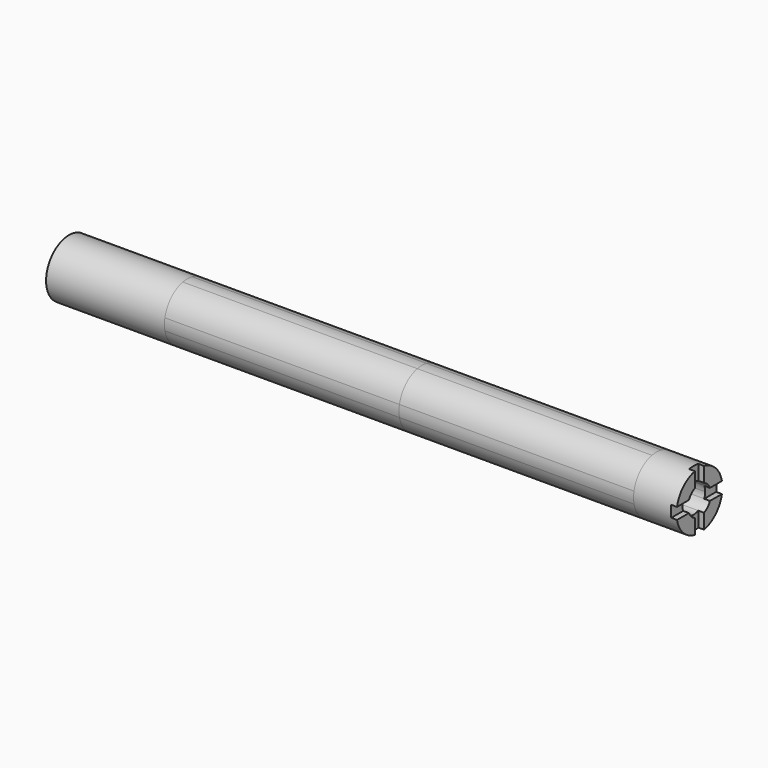
from build123d import *
from build123d import SkipClean  # not in build123d's __all__

# Parameters (mm, degrees)
F1_DEPTH  = 103.9495
F3_R      = 12.7
F4_DEPTH  = 19.05
F6_DEPTH  = 25.4
F8_DEPTH  = 2.54
F9_R      = 12.7
F10_DEPTH = 52.451


# Not quite as in the source:
# - after a boolean that leaves OpenCascade's solid faulty, fix() repairs it


with BuildPart() as f1:
    # F0 (on Right) → F1 (new body, symmetric)
    with BuildSketch(Plane.YZ):
        with BuildLine():
            ThreePointArc((12.4434078933, -2.54), (12.6356891432, -1.2764638175), (12.7, 0))
            ThreePointArc((12.7, 0), (12.6356891432, 1.2764638175), (12.4434078933, 2.54))
            Line((12.4434078933, 2.54), (5.8198711326, 2.54))
            ThreePointArc((5.8198711326, 2.54), (6.2160550871, 1.2973662374), (6.35, 0))
            ThreePointArc((6.35, 0), (6.2160550871, -1.2973662374), (5.8198711326, -2.54))
            Line((5.8198711326, -2.54), (12.4434078933, -2.54))
        make_face()
        with BuildLine():
            Line((5.8198711326, 2.54), (12.4434078933, 2.54))
            ThreePointArc((12.4434078933, 2.54), (8.9802561211, 8.9802561211), (2.54, 12.4434078933))
            Line((2.54, 12.4434078933), (2.54, 5.8198711326))
            ThreePointArc((2.54, 5.8198711326), (4.4901280605, 4.4901280605), (5.8198711326, 2.54))
        make_face()
        with BuildLine():
            ThreePointArc((2.54, -12.4434078933), (8.9802561211, -8.9802561211), (12.4434078933, -2.54))
            Line((12.4434078933, -2.54), (5.8198711326, -2.54))
            ThreePointArc((5.8198711326, -2.54), (4.4901280605, -4.4901280605), (2.54, -5.8198711326))
            Line((2.54, -5.8198711326), (2.54, -12.4434078933))
        make_face()
        with BuildLine():
            Line((2.54, 5.8198711326), (2.54, 12.4434078933))
            ThreePointArc((2.54, 12.4434078933), (0, 12.7), (-2.54, 12.4434078933))
            Line((-2.54, 12.4434078933), (-2.54, 5.8198711326))
            ThreePointArc((-2.54, 5.8198711326), (0, 6.35), (2.54, 5.8198711326))
        make_face()
        with BuildLine():
            ThreePointArc((-2.54, -12.4434078933), (0, -12.7), (2.54, -12.4434078933))
            Line((2.54, -12.4434078933), (2.54, -5.8198711326))
            ThreePointArc((2.54, -5.8198711326), (0, -6.35), (-2.54, -5.8198711326))
            Line((-2.54, -5.8198711326), (-2.54, -12.4434078933))
        make_face()
        with BuildLine():
            Line((-2.54, 5.8198711326), (-2.54, 12.4434078933))
            ThreePointArc((-2.54, 12.4434078933), (-8.9802561211, 8.9802561211), (-12.4434078933, 2.54))
            Line((-12.4434078933, 2.54), (-5.8198711326, 2.54))
            ThreePointArc((-5.8198711326, 2.54), (-4.4901280605, 4.4901280605), (-2.54, 5.8198711326))
        make_face()
        with BuildLine():
            ThreePointArc((-12.4434078933, -2.54), (-8.9802561211, -8.9802561211), (-2.54, -12.4434078933))
            Line((-2.54, -12.4434078933), (-2.54, -5.8198711326))
            ThreePointArc((-2.54, -5.8198711326), (-4.4901280605, -4.4901280605), (-5.8198711326, -2.54))
            Line((-5.8198711326, -2.54), (-12.4434078933, -2.54))
        make_face()
        with BuildLine():
            Line((-5.8198711326, 2.54), (-12.4434078933, 2.54))
            ThreePointArc((-12.4434078933, 2.54), (-12.7, 0), (-12.4434078933, -2.54))
            Line((-12.4434078933, -2.54), (-5.8198711326, -2.54))
            ThreePointArc((-5.8198711326, -2.54), (-6.35, 0), (-5.8198711326, 2.54))
        make_face()
        with BuildLine():
            ThreePointArc((6.35, 0), (6.2160550871, 1.2973662374), (5.8198711326, 2.54))
            ThreePointArc((5.8198711326, 2.54), (4.4901280605, 4.4901280605), (2.54, 5.8198711326))
            ThreePointArc((2.54, 5.8198711326), (0, 6.35), (-2.54, 5.8198711326))
            ThreePointArc((-2.54, 5.8198711326), (-4.4901280605, 4.4901280605), (-5.8198711326, 2.54))
            ThreePointArc((-5.8198711326, 2.54), (-6.35, 0), (-5.8198711326, -2.54))
            ThreePointArc((-5.8198711326, -2.54), (-4.4901280605, -4.4901280605), (-2.54, -5.8198711326))
            ThreePointArc((-2.54, -5.8198711326), (0, -6.35), (2.54, -5.8198711326))
            ThreePointArc((2.54, -5.8198711326), (4.4901280605, -4.4901280605), (5.8198711326, -2.54))
            ThreePointArc((5.8198711326, -2.54), (6.2160550871, -1.2973662374), (6.35, 0))
        make_face()
    extrude(amount=F1_DEPTH, both=True)

    # F3 (on face) → F4 (join)
    with BuildSketch(Plane.YZ.offset(103.9495)):
        Circle(F3_R)
    with SkipClean():  # cleaning this boolean's faces spoils the solid; the shape is the same uncleaned
        extrude(amount=F4_DEPTH)

    # F5 (on face) → F6 (cut)
    with BuildSketch(Plane.YZ.offset(122.9995)):
        with BuildLine():
            ThreePointArc((5.8198711326, -2.54), (6.2160550871, -1.2973662374), (6.35, 0))
            ThreePointArc((6.35, 0), (6.2160550871, 1.2973662374), (5.8198711326, 2.54))
            ThreePointArc((5.8198711326, 2.54), (4.4901280605, 4.4901280605), (2.54, 5.8198711326))
            ThreePointArc((2.54, 5.8198711326), (0, 6.35), (-2.54, 5.8198711326))
            ThreePointArc((-2.54, 5.8198711326), (-4.4901280605, 4.4901280605), (-5.8198711326, 2.54))
            ThreePointArc((-5.8198711326, 2.54), (-6.35, 0), (-5.8198711326, -2.54))
            ThreePointArc((-5.8198711326, -2.54), (-4.4901280605, -4.4901280605), (-2.54, -5.8198711326))
            ThreePointArc((-2.54, -5.8198711326), (0, -6.35), (2.54, -5.8198711326))
            ThreePointArc((2.54, -5.8198711326), (4.4901280605, -4.4901280605), (5.8198711326, -2.54))
        make_face()
    extrude(amount=-F6_DEPTH, mode=Mode.SUBTRACT)

    add(f1.part.fix(), mode=Mode.REPLACE)

    # F7 (on face) → F8 (cut)
    with BuildSketch(Plane.YZ.offset(122.9995)):
        with BuildLine():
            ThreePointArc((2.54, 12.4434078933), (0, 12.7), (-2.54, 12.4434078933))
            Line((-2.54, 12.4434078933), (-2.54, 5.8198711326))
            ThreePointArc((-2.54, 5.8198711326), (0, 6.35), (2.54, 5.8198711326))
            Line((2.54, 5.8198711326), (2.54, 12.4434078933))
        make_face()
        with BuildLine():
            ThreePointArc((12.7, 0), (12.6356891432, 1.2764638175), (12.4434078933, 2.54))
            Line((12.4434078933, 2.54), (5.8198711326, 2.54))
            ThreePointArc((5.8198711326, 2.54), (6.2160550871, 1.2973662374), (6.35, 0))
            ThreePointArc((6.35, 0), (6.2160550871, -1.2973662374), (5.8198711326, -2.54))
            Line((5.8198711326, -2.54), (12.4434078933, -2.54))
            ThreePointArc((12.4434078933, -2.54), (12.6356891432, -1.2764638175), (12.7, 0))
        make_face()
        with BuildLine():
            Line((-2.54, -5.8198711326), (-2.54, -12.4434078933))
            ThreePointArc((-2.54, -12.4434078933), (0, -12.7), (2.54, -12.4434078933))
            Line((2.54, -12.4434078933), (2.54, -5.8198711326))
            ThreePointArc((2.54, -5.8198711326), (0, -6.35), (-2.54, -5.8198711326))
        make_face()
        with BuildLine():
            Line((-5.8198711326, 2.54), (-12.4434078933, 2.54))
            ThreePointArc((-12.4434078933, 2.54), (-12.7, 0), (-12.4434078933, -2.54))
            Line((-12.4434078933, -2.54), (-5.8198711326, -2.54))
            ThreePointArc((-5.8198711326, -2.54), (-6.35, 0), (-5.8198711326, 2.54))
        make_face()
    extrude(amount=-F8_DEPTH, mode=Mode.SUBTRACT)

    # F9 (on face) → F10 (join)
    with BuildSketch(Plane(origin=(-103.9495, 0, 0), x_dir=(0, -1, 0), z_dir=(-1, 0, 0))):
        Circle(F9_R)
    with SkipClean():  # cleaning this boolean's faces spoils the solid; the shape is the same uncleaned
        extrude(amount=F10_DEPTH)


solid = f1.part
